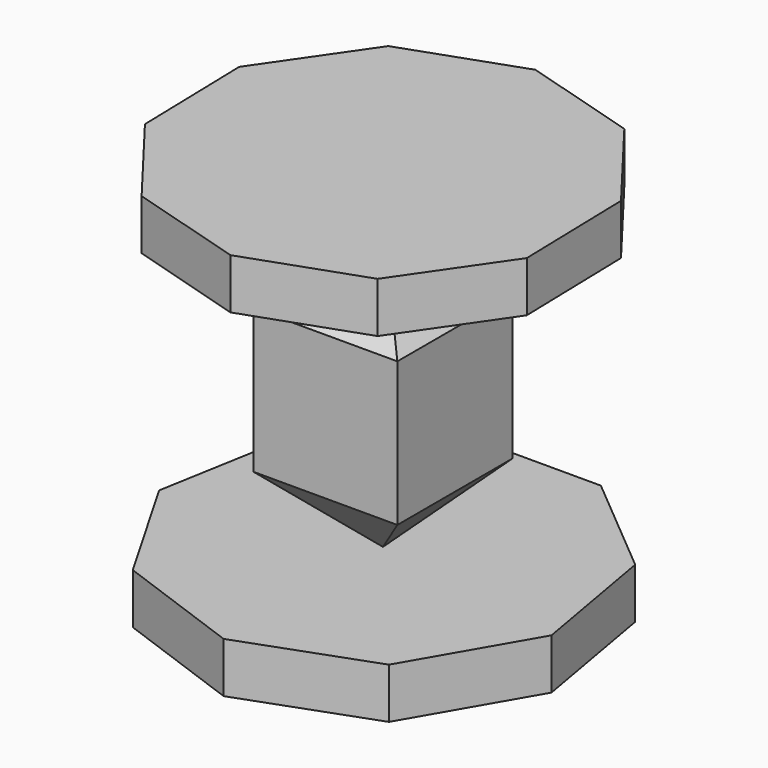
from build123d import *

# Parameters (mm, degrees)
F0_W      = 100
F0_H      = 100
F1_DEPTH  = 100
F2_DEPTH  = 50
F3_SIZE   = 49.99999
F6_DEPTH  = 35
F7_DEPTH  = 50
F8_SIZE   = 49.99999
F11_DEPTH = 35


# Not quite as in the source:
# - a fillet or chamfer is up to 0.001 mm smaller than in the source, because OpenCascade refuses the exact size


with BuildPart() as f1:
    # F0 (on Top) → F1 (new body)
    with BuildSketch(Plane.XY):
        Rectangle(F0_W, F0_H)
    extrude(amount=-F1_DEPTH)

    # F2 (add): a face of the model
    f2_faces = [f1.faces().sort_by_distance(p)[0] for p in [
        (0, 0, 0),
    ]]
    extrude(f2_faces, amount=F2_DEPTH)

    # F3 (size 50 in the source; OpenCascade refuses exactly that, so slightly less here)
    f3_edges = [f1.edges().sort_by_distance(p)[0] for p in [
        (0, -50, 50),
        (0, 50, 50),
        (50, 0, 50),
        (-50, 0, 50),
    ]]
    chamfer(f3_edges, length=F3_SIZE)

    # F7 (add): a face of the model
    f7_faces = [f1.faces().sort_by_distance(p)[0] for p in [
        (0, 0, -100),
    ]]
    extrude(f7_faces, amount=F7_DEPTH)

    # F8 (size 50 in the source; OpenCascade refuses exactly that, so slightly less here)
    f8_edges = [f1.edges().sort_by_distance(p)[0] for p in [
        (0, -50, -150),
        (50, 0, -150),
        (-50, 0, -150),
        (0, 50, -150),
    ]]
    chamfer(f8_edges, length=F8_SIZE)


with BuildPart() as f6:
    # F5 (on offset) → F6 (new body)
    with BuildSketch(Plane.XY.offset(50)):
        Polygon((83.0988892729, -108.5299731581), (131.0207312895, -38.9582910875), (128.8971071844, 45.494134035), (77.5391691864, 112.5693462448), (-3.4360959814, 136.6468942805), (-83.0988892729, 108.5299731581), (-131.0207312895, 38.9582910875), (-128.8971071844, -45.494134035), (-77.5391691864, -112.5693462448), (3.4360959814, -136.6468942805), align=None)
    extrude(amount=F6_DEPTH)


with BuildPart() as f11:
    # F10 (on offset) → F11 (new body)
    with BuildSketch(Plane.XY.offset(-150)):
        Polygon((47.3161304546, 130), (-47.3161304546, 130), (-119.8086480639, 69.1715552109), (-136.2413677193, -24.0230290175), (-88.9252372647, -105.9769709825), (0, -138.3431104219), (88.9252372647, -105.9769709825), (136.2413677193, -24.0230290175), (119.8086480639, 69.1715552109), align=None)
    extrude(amount=-F11_DEPTH)


solid = Compound([f1.part, f6.part, f11.part])
